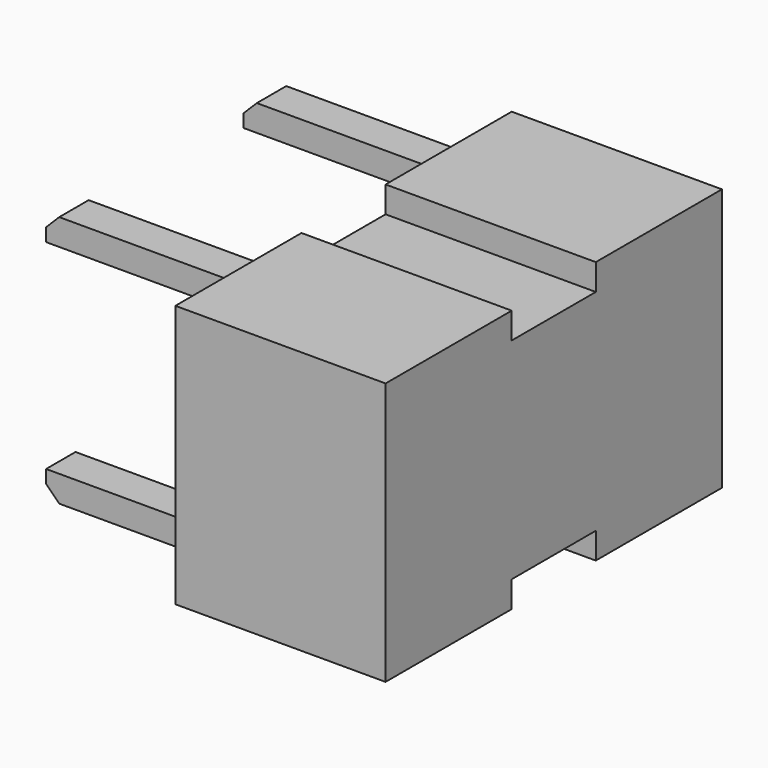
from build123d import *

# Parameters (mm, degrees)
F1_DEPTH = 50.8
F3_DEPTH = 8.89


with BuildPart() as f1:
    # F0 (on Right) → F1 (new body)
    with BuildSketch(Plane.YZ):
        Polygon((12.7, 25.4), (0, 25.4), (-12.7, 25.4), (-12.7, 31.75), (-50.8, 31.75), (-50.8, 0), (-50.8, -31.75), (-12.7, -31.75), (-12.7, -25.4), (0, -25.4), (12.7, -25.4), (12.7, -31.75), (50.8, -31.75), (50.8, 0), (50.8, 31.75), (12.7, 31.75), align=None)
    extrude(amount=F1_DEPTH)


with BuildPart() as f3:
    # F2 (on Front) → F3 (new body)
    with BuildSketch(Plane.XZ):
        Polygon((0, 19.05), (0, 25.4), (-41.275, 25.4), (-44.45, 22.225), (-44.45, 19.05), align=None)
    extrude(amount=F3_DEPTH)


with BuildPart() as f4_1:
    # F4: instance of F3
    add(f3.part.mirror(Plane.XY))


with BuildPart() as f3_1:
    # F5: moved
    add(f3.part.moved(Location((0, -38.1, 0))))


with BuildPart() as f4_1_1:
    # F5: moved
    add(f4_1.part.moved(Location((0, -38.1, 0))))


with BuildPart() as f3_2:
    # F6: moved
    add(f3_1.part.moved(Location((0, 0, 5.08))))


with BuildPart() as f4_1_2:
    # F7: moved
    add(f4_1_1.part.moved(Location((0, 0, -5.08))))


with BuildPart() as f8_1:
    # F8: instance of F3
    add(f3_2.part.mirror(Plane.XZ))


with BuildPart() as f8_2:
    # F8: instance of F4_1
    add(f4_1_2.part.mirror(Plane.XZ))


with BuildPart() as f3_3:
    # F9: moved
    add(f3_2.part.moved(Location((0, 12.7, 0))))


with BuildPart() as f4_1_3:
    # F9: moved
    add(f4_1_2.part.moved(Location((0, 12.7, 0))))


with BuildPart() as f8_1_1:
    # F10: moved
    add(f8_1.part.moved(Location((0, -12.7, 0))))


with BuildPart() as f8_2_1:
    # F10: moved
    add(f8_2.part.moved(Location((0, -12.7, 0))))


solid = Compound([f1.part, f3_3.part, f4_1_3.part, f8_1_1.part, f8_2_1.part])
